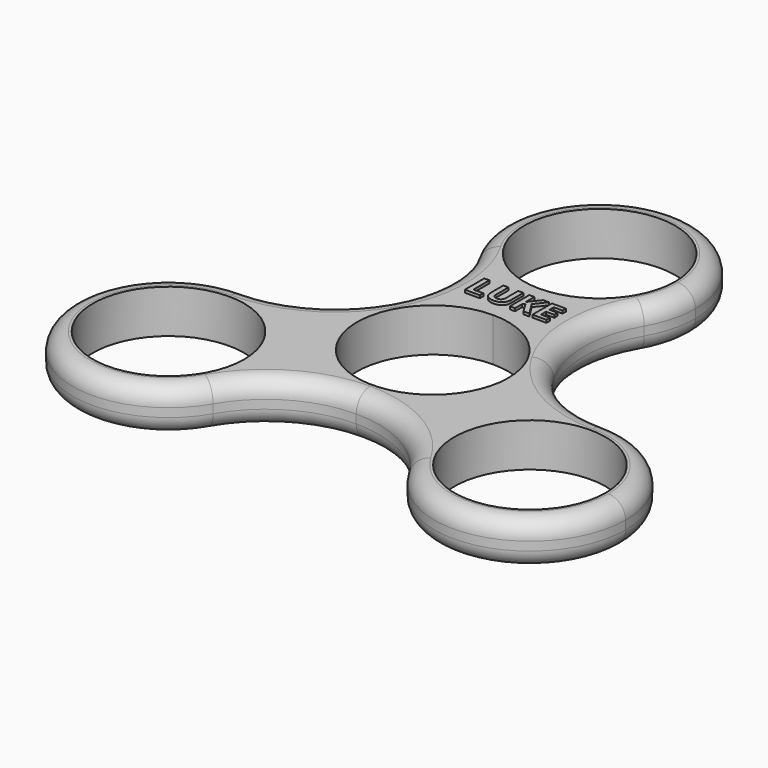
from build123d import *

# Parameters (mm, degrees)
F0_R         = 11.049
F1_DEPTH     = 6.35
F2_R         = 2.54
F3_TEXT_SIZE = 4.9788667688
F4_DEPTH     = 0.396875


# Not quite as in the source:
# - Text() gives the source's letters only with a copy of the font that has no kerning and outlines rounded to 1/6400 em; it was checked with that copy


with BuildPart() as f1:
    # F0 (on Top) → F1 (new body)
    with BuildSketch(Plane.XY):
        with BuildLine():
            ThreePointArc((0, 11.049), (7.8128228253, 7.8128228253), (11.049, 0))
            ThreePointArc((11.049, 0), (-2.8596916293, -10.6725144547), (-9.5687146864, 5.5245))
            Line((-9.5687146864, 5.5245), (-12.0983748909, 6.985))
            ThreePointArc((-12.0983748909, 6.985), (-12.0983748946, -6.9849999936), (-1.49e-08, -13.97))
            ThreePointArc((-1.49e-08, -13.97), (9.8782817279, -9.8782817384), (13.97, 0))
            ThreePointArc((13.97, 0), (13.4939838053, 3.6157020152), (12.0983749373, 6.9849999196))
            ThreePointArc((12.0983749373, 6.9849999196), (6.9850000402, 12.0983748677), (0, 13.97))
            Line((0, 13.97), (0, 11.049))
        make_face()
        with BuildLine():
            ThreePointArc((-9.5687146864, 5.5245), (-5.5245, 9.5687146864), (0, 11.049))
            Line((0, 11.049), (0, 13.97))
            ThreePointArc((0, 13.97), (-6.985, 12.0983748909), (-12.0983748909, 6.985))
            Line((-12.0983748909, 6.985), (-9.5687146864, 5.5245))
        make_face()
        with BuildLine():
            Line((0, 16.51), (0, 13.97))
            ThreePointArc((0, 13.97), (6.9850000402, 12.0983748677), (12.0983749373, 6.9849999196))
            ThreePointArc((12.0983749373, 6.9849999196), (9.8864543073, 15.2399999536), (12.0983748909, 23.495))
            ThreePointArc((12.0983748909, 23.495), (6.985, 18.3816251091), (0, 16.51))
        make_face()
        with BuildLine():
            ThreePointArc((-12.0983748909, 6.985), (-6.985, 12.0983748909), (0, 13.97))
            Line((0, 13.97), (0, 16.51))
            ThreePointArc((0, 16.51), (-6.985, 18.3816251091), (-12.0983748909, 23.495))
            ThreePointArc((-12.0983748909, 23.495), (-9.8864543073, 15.24), (-12.0983748909, 6.985))
        make_face()
        with BuildLine():
            ThreePointArc((-1.49e-08, -13.97), (-12.0983748946, -6.9849999936), (-12.0983748909, 6.985))
            ThreePointArc((-12.0983748909, 6.985), (-18.1414543073, 0.9419205835), (-26.3964543073, -1.27))
            ThreePointArc((-26.3964543073, -1.27), (-16.5181725742, -5.3617182668), (-12.4264543073, -15.24))
            ThreePointArc((-12.4264543073, -15.24), (-12.9024705141, -18.8557020601), (-14.2980794165, -22.225))
            ThreePointArc((-14.2980794165, -22.225), (-8.2550000064, -16.1819205872), (-1.49e-08, -13.97))
        make_face()
        with BuildLine():
            ThreePointArc((26.3964543073, -1.27), (18.1414543475, 0.9419205603), (12.0983749373, 6.9849999196))
            ThreePointArc((12.0983749373, 6.9849999196), (13.4939838053, 3.6157020152), (13.97, 0))
            ThreePointArc((13.97, 0), (9.8782817279, -9.8782817384), (-1.49e-08, -13.97))
            ThreePointArc((-1.49e-08, -13.97), (8.2549999936, -16.1819205798), (14.2980794165, -22.225))
            ThreePointArc((14.2980794165, -22.225), (14.2980794165, -8.255), (26.3964543073, -1.27))
        make_face()
        with BuildLine():
            ThreePointArc((-12.0983748909, 23.495), (-6.985, 18.3816251091), (0, 16.51))
            ThreePointArc((0, 16.51), (6.985, 18.3816251091), (12.0983748909, 23.495))
            ThreePointArc((12.0983748909, 23.495), (13.4939837933, 26.8642979399), (13.97, 30.48))
            ThreePointArc((13.97, 30.48), (-3.6157020601, 43.9739837933), (-12.0983748909, 23.495))
        make_face()
        with BuildLine():
            ThreePointArc((11.049, 30.48), (7.8128228253, 22.6671771747), (0, 19.431))
            ThreePointArc((0, 19.431), (-7.8128228253, 38.2928228253), (11.049, 30.48))
        make_face(mode=Mode.SUBTRACT)
        with BuildLine():
            ThreePointArc((-12.4264543073, -15.24), (-16.5181725742, -5.3617182668), (-26.3964543073, -1.27))
            ThreePointArc((-26.3964543073, -1.27), (-38.4948291982, -22.225), (-14.2980794165, -22.225))
            ThreePointArc((-14.2980794165, -22.225), (-12.9024705141, -18.8557020601), (-12.4264543073, -15.24))
        make_face()
        with Locations((-26.3964543073, -15.24)):
            Circle(F0_R, mode=Mode.SUBTRACT)
        with BuildLine():
            ThreePointArc((40.3664543073, -15.24), (36.2747360405, -5.3617182668), (26.3964543073, -1.27))
            ThreePointArc((26.3964543073, -1.27), (14.2980794165, -8.255), (14.2980794165, -22.225))
            ThreePointArc((14.2980794165, -22.225), (30.0121563674, -28.7339837933), (40.3664543073, -15.24))
        make_face()
        with Locations((26.3964543073, -15.24)):
            Circle(F0_R, mode=Mode.SUBTRACT)
    extrude(amount=F1_DEPTH)

    # F2
    f2_edges = [f1.edges().sort_by_distance(p)[0] for p in [
        (0, -13.97, 6.35),
        (-12.098375, 6.985, 0),
        (-12.098375, 6.985, 6.35),
        (-38.494829, -22.225, 0),
        (-38.494829, -22.225, 6.35),
        (0, -13.97, 0),
        (38.494829, -22.225, 0),
        (38.494829, -22.225, 6.35),
        (12.098375, 6.985, 0),
        (12.098375, 6.985, 6.35),
        (0, 44.45, 0),
        (0, 44.45, 6.35),
    ]]
    fillet(f2_edges, radius=F2_R)

    # F3 (on face) → F4 (join)
    with BuildSketch(Plane.XY.offset(6.35)):
        with Locations((-6.4244154455, 13.3339520601)):
            Text('LUKE', F3_TEXT_SIZE, font='Open Sans', font_style=FontStyle.BOLD, text_align=(TextAlign.LEFT, TextAlign.BOTTOM))
    extrude(amount=F4_DEPTH)


solid = f1.part
